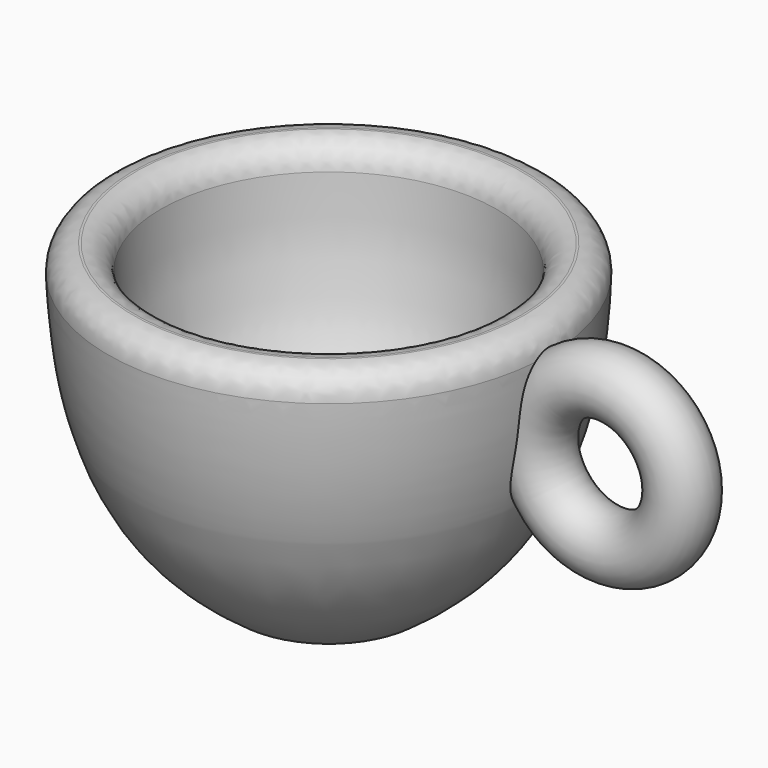
from build123d import *

# Parameters (mm, degrees)
F2_T = -3.175
F3_R = 1.524
F6_R = 1.8631814182
F8_R = 5.08


with BuildPart() as f1:
    # F0 (on Front) → F1 (revolve)
    with BuildSketch(Plane.XZ):
        with BuildLine():
            Line((0, 18.6147112399), (0, 0))
            Line((0, 0), (4.9660643563, 0))
            add(Edge.make_bspline(
                [(4.9660643563, 0), (8.8066002354, 2.6415751781), (13.2581302896, 6.4821103588), (13.2581302896, 18.6147112399)],
                knots=[0, 0, 0, 0, 20.3780723325, 20.3780723325, 20.3780723325, 20.3780723325], degree=3))
            Line((13.2581302896, 18.6147112399), (0, 18.6147112399))
        make_face()
    revolve(axis=Axis((0, 0, -0.4398934543), (0, 0, -1)))

    # F2
    f2_openings = [f1.faces().sort_by_distance(p)[0] for p in [
        (0, 0, 18.614711),
    ]]
    offset(amount=F2_T, openings=f2_openings)

    # F3
    f3_edges = [f1.edges().sort_by_distance(p)[0] for p in [
        (-13.25813, 0, 18.614711),
        (-4.966064, 0, 0),
        (-10.08313, 0, 18.614711),
    ]]
    fillet(f3_edges, radius=F3_R)

    # F7: sweep along a path in F4
    with BuildLine(Plane.XZ) as f7_path:
        CenterArc((16.8713424355, 12.4752419069), 5.1659744209, 0, 360)
    # F6 (on line) → F7 (sweep)
    with BuildSketch(Plane(origin=(0, 0, 12.4752419069), x_dir=(1, 0, 0), z_dir=(0, 0, -1))):
        with Locations((21.1782623082, 0)):
            Circle(F6_R)
    sweep(path=f7_path.line)

    # F8
    f8_edges = [f1.edges().sort_by_distance(p)[0] for p in [
        (-3.956802, 0, 3.175),
    ]]
    fillet(f8_edges, radius=F8_R)


solid = f1.part
